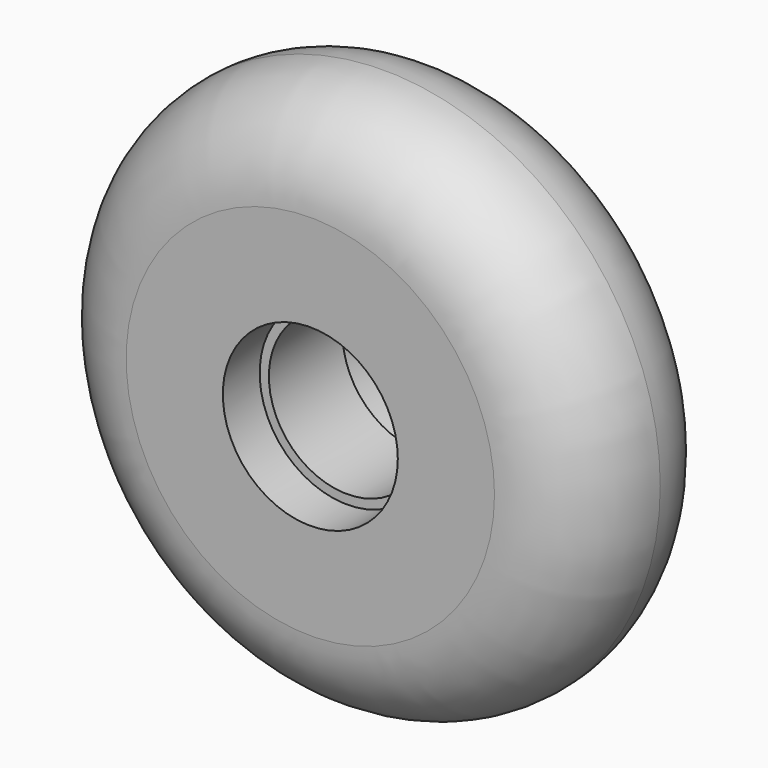
from build123d import *

# Parameters (mm, degrees)
F0_R     = 38.1
F1_DEPTH = 12.7
F2_R     = 12.69999
F3_R     = 10.795
F4_DEPTH = 25.4
F6_R     = 12.065
F7_DEPTH = 6.35


# Not quite as in the source:
# - a fillet or chamfer is up to 0.001 mm smaller than in the source, because OpenCascade refuses the exact size


with BuildPart() as f1:
    # F0 (on Front) → F1 (new body)
    with BuildSketch(Plane.XZ):
        Circle(F0_R)
    extrude(amount=F1_DEPTH)

    # F2 (radius 12.7 in the source; OpenCascade refuses exactly that, so slightly less here)
    f2_edges = [f1.edges().sort_by_distance(p)[0] for p in [
        (-38.1, -12.7, 0),
    ]]
    fillet(f2_edges, radius=F2_R)

    # F3 (on Front) → F4 (cut)
    with BuildSketch(Plane.XZ):
        Circle(F3_R)
    extrude(amount=F4_DEPTH, mode=Mode.SUBTRACT)

    # F6 (on offset) → F7 (cut)
    with BuildSketch(Plane.XZ.offset(12.7)):
        Circle(F6_R)
    extrude(amount=-F7_DEPTH, mode=Mode.SUBTRACT)

    # F8: F1 across plane


with BuildPart() as f1_1:
    add(f1.part)
    add(f1.part.mirror(Plane.XZ))


solid = f1_1.part
